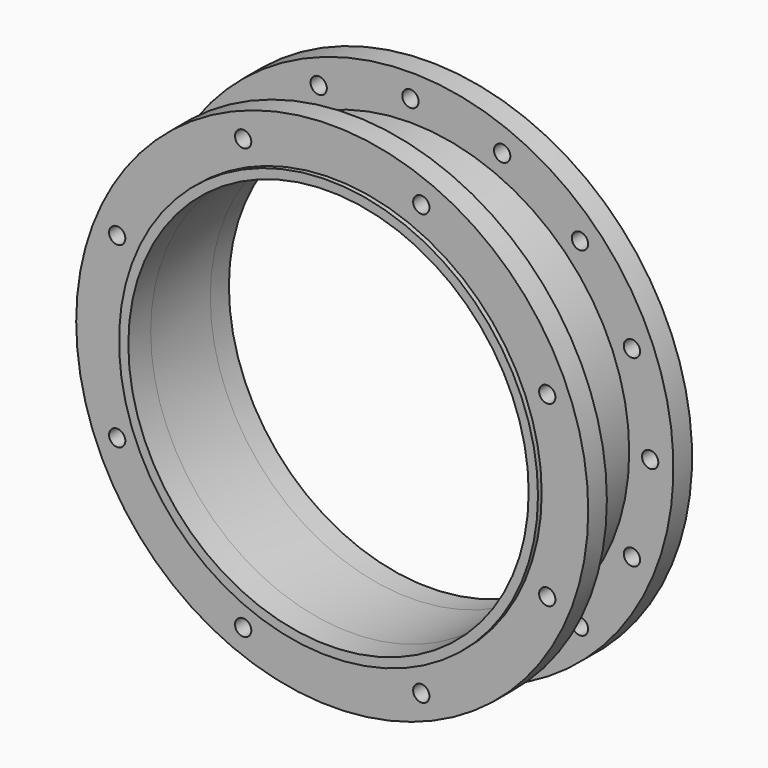
from build123d import *
from build123d import SkipClean  # not in build123d's __all__

# Parameters (mm, degrees)
F0_R             = 275
F1_DEPTH         = 25
F3_D             = 17.5
F3_COPIES_COUNT  = 8
F4_R             = 225
F5_DEPTH         = 5
F6_R             = 215
F7_DEPTH         = 30.001
F8_R             = 235
F8_R_2           = 215
F9_DEPTH         = 80
F10_R            = 282.5
F10_R_2          = 235
F10_R_3          = 215
F11_DEPTH        = 25
F13_D            = 17.5
F13_DEPTH        = 25
F13_TIP          = 5.2575304165
F13_COPIES_COUNT = 16


# Not quite as in the source:
# - after a boolean that leaves OpenCascade's solid faulty, fix() repairs it
# - a pattern or mirror of a feature is missing from the dataset's text; its kind, count and spacing are read off the source's solid


with BuildPart() as f1:
    # F0 (on Front) → F1 (new body)
    with BuildSketch(Plane.XZ):
        Circle(F0_R)
    extrude(amount=F1_DEPTH)

    # F3 (through all)
    with Locations(Plane.XZ.offset(25)):
        with Locations((95.6708580913, 230.9698831278)):
            f3 = Hole(F3_D / 2)

    # F3_copies: F3 ×8 about axis
    f3_copies_axis = Axis((0, 0, 0), (0, 1, 0))
    for i in range(1, F3_COPIES_COUNT):
        add(f3.rotate(f3_copies_axis, i * 360 / F3_COPIES_COUNT), clean=False, mode=Mode.SUBTRACT)

    # F4 (on face) → F5 (join)
    with BuildSketch(Plane.XZ.offset(25)):
        Circle(F4_R)
    extrude(amount=F5_DEPTH)

    # F6 (on face) → F7 (cut, through all)
    with BuildSketch(Plane.XZ.offset(30)):
        Circle(F6_R)
    extrude(amount=-F7_DEPTH, mode=Mode.SUBTRACT)

    # F8 (on face) → F9 (join)
    with BuildSketch(Plane(origin=(0, 0, 0), x_dir=(-1, 0, 0), z_dir=(0, 1, 0))):
        Circle(F8_R)
        Circle(F8_R_2, mode=Mode.SUBTRACT)
    with SkipClean():  # cleaning this boolean's faces spoils the solid; the shape is the same uncleaned
        extrude(amount=F9_DEPTH)

    # F10 (on face) → F11 (join)
    with BuildSketch(Plane(origin=(0, 80, 0), x_dir=(-1, 0, 0), z_dir=(0, 1, 0))):
        Circle(F10_R)
        Circle(F10_R_2, mode=Mode.SUBTRACT)
        Circle(F10_R_2)
        Circle(F10_R_3, mode=Mode.SUBTRACT)
    extrude(amount=F11_DEPTH)

    add(f1.part.fix(), mode=Mode.REPLACE)

    # F13
    with Locations(Plane(origin=(0, 105, 0), x_dir=(-1, 0, 0), z_dir=(0, 1, 0))):
        with Locations((0, 257.5)):
            f13 = Hole(F13_D / 2, depth=F13_DEPTH)
            with Locations((0, 0, -(F13_DEPTH + F13_TIP / 2))):  # 118° drill point
                Cone(0, F13_D / 2, F13_TIP, mode=Mode.SUBTRACT)

    # F13_copies: F13 ×16 about axis
    f13_copies_axis = Axis((0, 0, 0), (0, 1, 0))
    for i in range(1, F13_COPIES_COUNT):
        add(f13.rotate(f13_copies_axis, i * 360 / F13_COPIES_COUNT), clean=False, mode=Mode.SUBTRACT)


solid = f1.part
